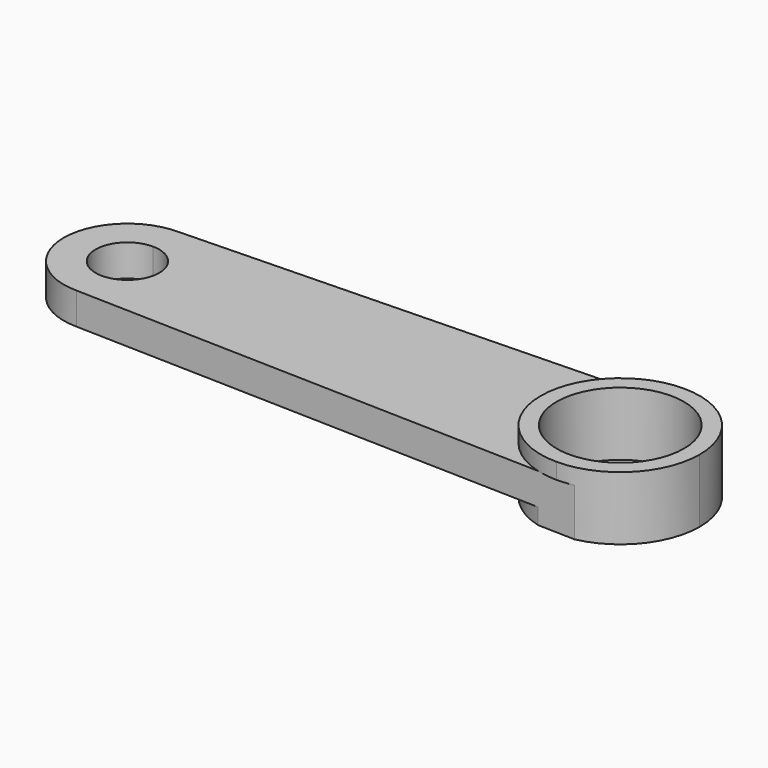
from build123d import *
from build123d import SkipClean  # not in build123d's __all__

# Parameters (mm, degrees)
F0_W          = 25.4
F0_H          = 6.35
F1_DEPTH      = 1.27
F4_DEPTH      = 25.4
F6_DEPTH      = 0.635
F6_DEPTH_BACK = 1.905
F7_R          = 2.54
F8_DEPTH      = 25.4
F9_DEPTH      = 25.4


with BuildPart() as f1:
    # F0 (on Top) → F1 (new body)
    with BuildSketch(Plane.XY):
        Rectangle(F0_W, F0_H)
    extrude(amount=F1_DEPTH)

    # F3 (on face) → F4 (cut)
    with BuildSketch(Plane.XY.offset(1.27)):
        with BuildLine():
            Line((12.7, -3.175), (12.7, 0))
            ThreePointArc((12.7, 0), (11.770064, -2.245064), (9.525, -3.175))
            Line((9.525, -3.175), (12.7, -3.175))
        make_face()
        with BuildLine():
            ThreePointArc((9.525, 3.175), (11.770064, 2.245064), (12.7, 0))
            Line((12.7, 0), (12.7, 3.175))
            Line((12.7, 3.175), (9.525, 3.175))
        make_face()
    extrude(amount=-F4_DEPTH, mode=Mode.SUBTRACT)

    # F5 (on face) → F6 (join, two sides)
    with BuildSketch(Plane.XY.offset(1.27)) as f6_sk:
        with BuildLine():
            ThreePointArc((9.525, -3.175), (11.770064, -2.245064), (12.7, 0))
            ThreePointArc((12.7, 0), (11.770064, 2.245064), (9.525, 3.175))
            ThreePointArc((9.525, 3.175), (6.35, 0), (9.525, -3.175))
        make_face()
    with SkipClean():  # cleaning this boolean's faces spoils the solid; the shape is the same uncleaned
        extrude(amount=F6_DEPTH)
        extrude(f6_sk.sketch, amount=-F6_DEPTH_BACK)

    # F7 (on face) → F8 (cut)
    with BuildSketch(Plane.XY.offset(1.905)):
        with Locations((9.525, 0)):
            Circle(F7_R)
    extrude(amount=-F8_DEPTH, mode=Mode.SUBTRACT)

    # F2 (on face) → F9 (cut)
    with BuildSketch(Plane.XY.offset(1.27)):
        with BuildLine():
            Line((12.7, -3.175), (-10.16, -2.54))
            ThreePointArc((-10.16, -2.54), (-11.956051, -1.796051), (-12.7, 0))
            Line((-12.7, 0), (-12.7, -3.175))
            Line((-12.7, -3.175), (12.7, -3.175))
        make_face()
        with BuildLine():
            ThreePointArc((-12.7, 0), (-11.956051, 1.796051), (-10.16, 2.54))
            Line((-10.16, 2.54), (12.7, 3.175))
            Line((12.7, 3.175), (-12.7, 3.175))
            Line((-12.7, 3.175), (-12.7, 0))
        make_face()
        with BuildLine():
            ThreePointArc((-8.89, 0), (-9.261974, 0.898026), (-10.16, 1.27))
            Line((-10.16, 1.27), (-10.16, 0))
            Line((-10.16, 0), (-10.16, -1.27))
            ThreePointArc((-10.16, -1.27), (-9.261974, -0.898026), (-8.89, 0))
        make_face()
        with BuildLine():
            Line((-10.16, 0), (-10.16, 1.27))
            ThreePointArc((-10.16, 1.27), (-11.43, 0), (-10.16, -1.27))
            Line((-10.16, -1.27), (-10.16, 0))
        make_face()
    extrude(amount=-F9_DEPTH, mode=Mode.SUBTRACT)


solid = f1.part
